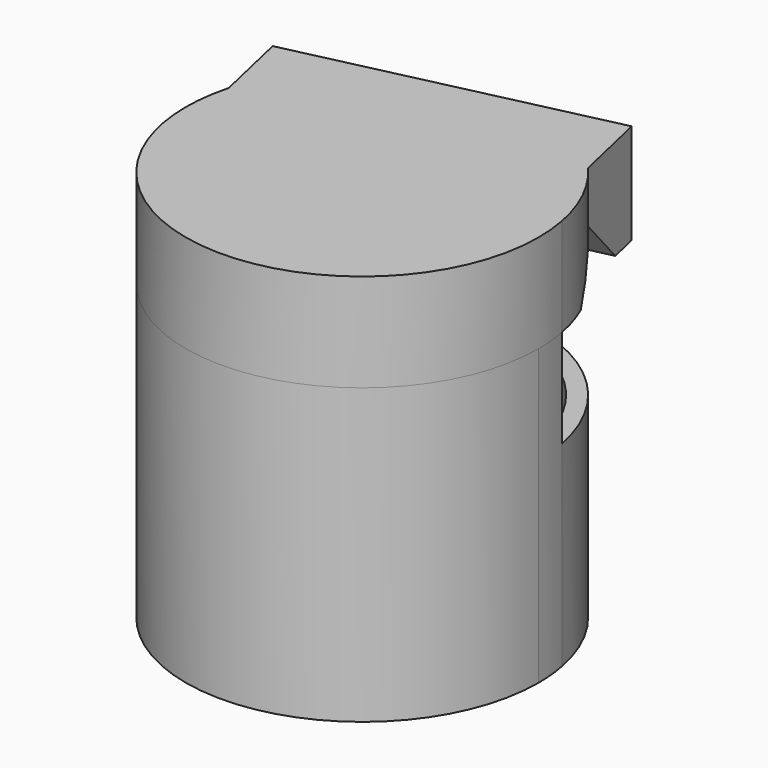
from build123d import *

# Parameters (mm, degrees)
F1_DEPTH = 30
F2_DEPTH = 20
F4_DEPTH = 10
F5_SIZE  = 5
F6_W     = 31.7785144259
F6_H     = 10.2327512205
F6_H_2   = 5
F7_DEPTH = 8
F8_SIZE  = 5


with BuildPart() as f1:
    # F0 (on Top) → F1 (new body)
    with BuildSketch(Plane.XY):
        with BuildLine():
            ThreePointArc((15.9804643873, 2.9474154722), (16.182475804, 1.4798570381), (16.25, 0))
            ThreePointArc((16.25, 0), (2.1533060737, -16.1066996294), (-15.6793259019, -4.2686343556))
            Line((-15.6793259019, -4.2686343556), (-17.3869081956, -4.6578346252))
            ThreePointArc((-17.3869081956, -4.6578346252), (2.3490053723, -17.8460688601), (18, 0))
            ThreePointArc((18, 0), (17.9218419848, 1.6755834418), (17.6880466811, 3.3366157419))
            Line((17.6880466811, 3.3366157419), (15.9804643873, 2.9474154722))
        make_face()
    extrude(amount=F1_DEPTH)

    # F0 (on Top) → F2 (join)
    with BuildSketch(Plane.XY):
        with BuildLine():
            ThreePointArc((15.9804643873, 2.9474154722), (16.182475804, 1.4798570381), (16.25, 0))
            ThreePointArc((16.25, 0), (2.1533060737, -16.1066996294), (-15.6793259019, -4.2686343556))
            Line((-15.6793259019, -4.2686343556), (-17.3869081956, -4.6578346252))
            ThreePointArc((-17.3869081956, -4.6578346252), (2.3490053723, -17.8460688601), (18, 0))
            ThreePointArc((18, 0), (17.9218419848, 1.6755834418), (17.6880466811, 3.3366157419))
            Line((17.6880466811, 3.3366157419), (15.9804643873, 2.9474154722))
        make_face()
        with BuildLine():
            ThreePointArc((-15.6793259019, -4.2686343556), (-3.6111653073, 15.8436733469), (15.9804643873, 2.9474154722))
            Line((15.9804643873, 2.9474154722), (17.6880466811, 3.3366157419))
            ThreePointArc((17.6880466811, 3.3366157419), (-4.0000600327, 17.549915092), (-17.3869081956, -4.6578346252))
            Line((-17.3869081956, -4.6578346252), (-15.6793259019, -4.2686343556))
        make_face()
    extrude(amount=F2_DEPTH)

    # F3 (on face) → F4 (join)
    with BuildSketch(Plane.XY.offset(30)):
        with BuildLine():
            ThreePointArc((15.9804643873, 2.9474154722), (3.6111653073, -15.8436733469), (-15.6793259019, -4.2686343556))
            Line((-15.6793259019, -4.2686343556), (-17.3869081956, -4.6578346252))
            ThreePointArc((-17.3869081956, -4.6578346252), (4.0000600327, -17.549915092), (17.6880466811, 3.3366157419))
            Line((17.6880466811, 3.3366157419), (15.9804643873, 2.9474154722))
        make_face()
        with BuildLine():
            Line((-17.3869081956, -4.6578346252), (-15.6793259019, -4.2686343556))
            ThreePointArc((-15.6793259019, -4.2686343556), (3.6111653073, -15.8436733469), (15.9804643873, 2.9474154722))
            Line((15.9804643873, 2.9474154722), (17.6880466811, 3.3366157419))
            ThreePointArc((17.6880466811, 3.3366157419), (16.2041492949, 7.8374450957), (13.5969934668, 11.7949891337))
            Line((13.5969934668, 11.7949891337), (-17.3652541608, 4.7379265435))
            ThreePointArc((-17.3652541608, 4.7379265435), (-17.3761273243, 4.6978930607), (-17.3869081956, 4.6578346252))
            ThreePointArc((-17.3869081956, 4.6578346252), (-17.9872433705, 0.6775514234), (-17.6880466811, -3.3366157419))
            Line((-17.6880466811, -3.3366157419), (-17.3869081956, -4.6578346252))
        make_face()
        with BuildLine():
            Line((-17.3869081956, 4.732991053), (-17.3869081956, 4.6578346252))
            ThreePointArc((-17.3869081956, 4.6578346252), (-17.3761273243, 4.6978930607), (-17.3652541608, 4.7379265435))
            Line((-17.3652541608, 4.7379265435), (-17.3869081956, 4.732991053))
        make_face()
    extrude(amount=F4_DEPTH)

    # F5
    f5_edges = [f1.edges().sort_by_distance(p)[0] for p in [
        (-1.894957, 8.26399, 30),
    ]]
    chamfer(f5_edges, length=F5_SIZE)

    # F6 (on face) → F7 (join)
    with BuildSketch(Plane(origin=(-1.884130347, 8.2664578386, 0), x_dir=(-0.9749952829, -0.2222255574, 0), z_dir=(-0.2222255574, 0.9749952829, 0))):
        with Locations((0.011104687, 34.8836243898)):
            Rectangle(F6_W, F6_H)
        with Locations((0.011104687, 37.5)):
            Rectangle(F6_W, F6_H_2)
    extrude(amount=F7_DEPTH)

    # F8
    f8_edges = [f1.edges().sort_by_distance(p)[0] for p in [
        (-1.894957, 8.26399, 29.767249),
    ]]
    chamfer(f8_edges, length=F8_SIZE)


solid = f1.part
